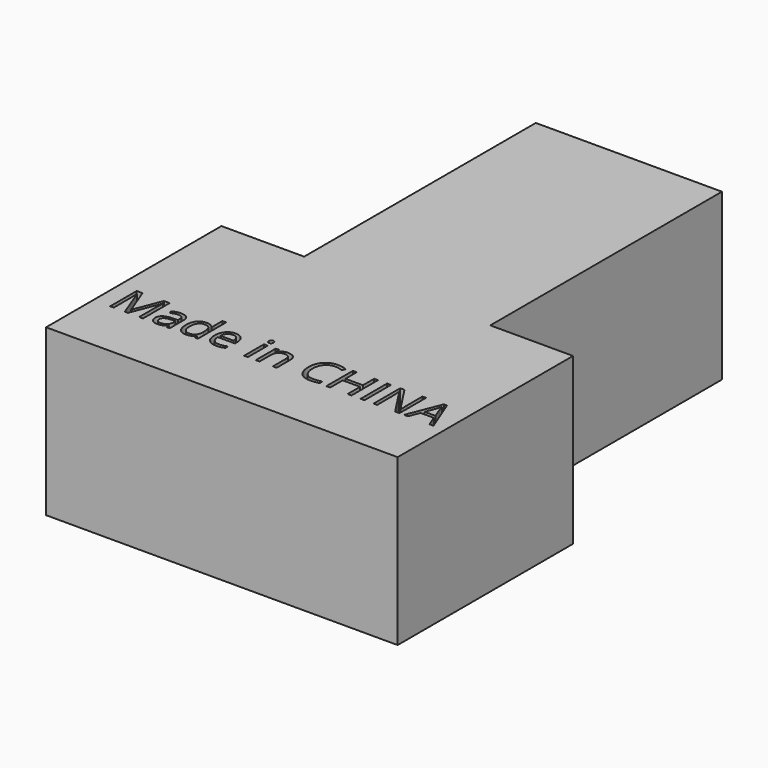
from build123d import *

# Parameters (mm, degrees)
F0_W         = 2.3149197708
F0_H         = 15.276686349
F0_W_2       = 2.3684439274
F0_H_2       = 20.3793226068
F0_W_3       = 114.3
F0_H_3       = 177.8
F0_TEXT_SIZE = 28.5462168273
F1_DEPTH     = 101.6
F2_DEPTH     = 254


# Not quite as in the source:
# - Text() gives the source's letters only with a copy of the font that has no kerning and outlines rounded to 1/6400 em; it was checked with that copy


with BuildPart() as f1:
    # F0 (on Top) → F1 (new body)
    with BuildSketch(Plane.XY):
        Polygon((-51.415306741, 48.4471506375), (-102.215306741, 48.4471506375), (-102.215306741, -86.1728493625), (113.684693259, -86.1728493625), (113.684693259, 48.4471506375), (62.884693259, 48.4471506375), align=None)
        with BuildLine():
            Line((-80.9077623426, -49.9574655533), (-82.816790593, -49.9574655533))
            Line((-82.816790593, -49.9574655533), (-89.7303274808, -31.8930627173))
            Line((-89.7303274808, -31.8930627173), (-89.8418361403, -31.8930627173))
            add(Edge.make_bspline(
                [(-89.8418361403, -31.8930627173), (-89.6455808996, -34.0384893257), (-89.6455808996, -36.9956989751)],
                knots=[0, 0, 0, 1, 1, 1], degree=2))
            Line((-89.6455808996, -36.9956989751), (-89.6455808996, -49.9574655533))
            Line((-89.6455808996, -49.9574655533), (-91.8356109718, -49.9574655533))
            Line((-91.8356109718, -49.9574655533), (-91.8356109718, -29.5781429464))
            Line((-91.8356109718, -29.5781429464), (-88.2673338684, -29.5781429464))
            Line((-88.2673338684, -29.5781429464), (-81.8132126576, -46.3891884499))
            Line((-81.8132126576, -46.3891884499), (-81.7017039981, -46.3891884499))
            Line((-81.7017039981, -46.3891884499), (-75.1940586308, -29.5781429464))
            Line((-75.1940586308, -29.5781429464), (-71.6525436057, -29.5781429464))
            Line((-71.6525436057, -29.5781429464), (-71.6525436057, -49.9574655533))
            Line((-71.6525436057, -49.9574655533), (-74.0209875331, -49.9574655533))
            Line((-74.0209875331, -49.9574655533), (-74.0209875331, -36.8262058127))
            add(Edge.make_bspline(
                [(-74.0209875331, -36.8262058127), (-74.0209875331, -34.5692705448), (-73.8247322924, -31.9198247955)],
                knots=[0, 0, 0, 1, 1, 1], degree=2))
            Line((-73.8247322924, -31.9198247955), (-73.9362409518, -31.9198247955))
            Line((-73.9362409518, -31.9198247955), (-80.9077623426, -49.9574655533))
        make_face(mode=Mode.SUBTRACT)
        with BuildLine():
            Line((-55.3009137793, -49.9574655533), (-57.0181471353, -49.9574655533))
            Line((-57.0181471353, -49.9574655533), (-57.4775628124, -47.7808165202))
            Line((-57.4775628124, -47.7808165202), (-57.5890714719, -47.7808165202))
            add(Edge.make_bspline(
                [(-57.5890714719, -47.7808165202), (-58.7309201449, -49.2170480543), (-59.8660782985, -49.7277577147)],
                knots=[0, 0, 0, 1, 1, 1], degree=2))
            add(Edge.make_bspline(
                [(-59.8660782985, -49.7277577147), (-61.001236452, -50.2384673752), (-62.7050887689, -50.2384673752)],
                knots=[0, 0, 0, 1, 1, 1], degree=2))
            add(Edge.make_bspline(
                [(-62.7050887689, -50.2384673752), (-64.9754050759, -50.2384673752), (-66.2644451795, -49.0653962774)],
                knots=[0, 0, 0, 1, 1, 1], degree=2))
            add(Edge.make_bspline(
                [(-66.2644451795, -49.0653962774), (-67.5534852831, -47.8923251797), (-67.5534852831, -45.7335175321)],
                knots=[0, 0, 0, 1, 1, 1], degree=2))
            add(Edge.make_bspline(
                [(-67.5534852831, -45.7335175321), (-67.5534852831, -41.1081383368), (-60.1537706399, -40.8851210178)],
                knots=[0, 0, 0, 1, 1, 1], degree=2))
            Line((-60.1537706399, -40.8851210178), (-57.5623093936, -40.8003744366))
            Line((-57.5623093936, -40.8003744366), (-57.5623093936, -39.8503206579))
            add(Edge.make_bspline(
                [(-57.5623093936, -39.8503206579), (-57.5623093936, -38.052801067), (-58.3339493172, -37.1964145622)],
                knots=[0, 0, 0, 1, 1, 1], degree=2))
            add(Edge.make_bspline(
                [(-58.3339493172, -37.1964145622), (-59.1055892408, -36.3400280574), (-60.8094415577, -36.3400280574)],
                knots=[0, 0, 0, 1, 1, 1], degree=2))
            add(Edge.make_bspline(
                [(-60.8094415577, -36.3400280574), (-62.718469808, -36.3400280574), (-65.1270568528, -37.5086388087)],
                knots=[0, 0, 0, 1, 1, 1], degree=2))
            Line((-65.1270568528, -37.5086388087), (-65.8407122735, -35.7378812962))
            add(Edge.make_bspline(
                [(-65.8407122735, -35.7378812962), (-64.7122446395, -35.1268138422), (-63.3674502062, -34.7789068246)],
                knots=[0, 0, 0, 1, 1, 1], degree=2))
            add(Edge.make_bspline(
                [(-63.3674502062, -34.7789068246), (-62.0226557728, -34.4309998071), (-60.6667104735, -34.4309998071)],
                knots=[0, 0, 0, 1, 1, 1], degree=2))
            add(Edge.make_bspline(
                [(-60.6667104735, -34.4309998071), (-57.9369784894, -34.4309998071), (-56.6189461344, -35.641983849)],
                knots=[0, 0, 0, 1, 1, 1], degree=2))
            add(Edge.make_bspline(
                [(-56.6189461344, -35.641983849), (-55.3009137793, -36.852967891), (-55.3009137793, -39.5291757186)],
                knots=[0, 0, 0, 1, 1, 1], degree=2))
            Line((-55.3009137793, -39.5291757186), (-55.3009137793, -49.9574655533))
        make_face(mode=Mode.SUBTRACT)
        with BuildLine():
            Line((-39.832432536, -49.9574655533), (-40.1401964362, -47.9101665652))
            Line((-40.1401964362, -47.9101665652), (-40.2650861348, -47.9101665652))
            add(Edge.make_bspline(
                [(-40.2650861348, -47.9101665652), (-41.866350485, -50.2384673752), (-45.0599584925, -50.2384673752)],
                knots=[0, 0, 0, 1, 1, 1], degree=2))
            add(Edge.make_bspline(
                [(-45.0599584925, -50.2384673752), (-48.0573112594, -50.2384673752), (-49.723250632, -48.1889382139)],
                knots=[0, 0, 0, 1, 1, 1], degree=2))
            add(Edge.make_bspline(
                [(-49.723250632, -48.1889382139), (-51.3891900047, -46.1394090526), (-51.3891900047, -42.3614956694)],
                knots=[0, 0, 0, 1, 1, 1], degree=2))
            add(Edge.make_bspline(
                [(-51.3891900047, -42.3614956694), (-51.3891900047, -38.5835822861), (-49.7165601125, -36.4916798343)],
                knots=[0, 0, 0, 1, 1, 1], degree=2))
            add(Edge.make_bspline(
                [(-49.7165601125, -36.4916798343), (-48.0439302202, -34.3997773824), (-45.0599584925, -34.3997773824)],
                knots=[0, 0, 0, 1, 1, 1], degree=2))
            add(Edge.make_bspline(
                [(-45.0599584925, -34.3997773824), (-41.9510970662, -34.3997773824), (-40.2918482131, -36.6611729967)],
                knots=[0, 0, 0, 1, 1, 1], degree=2))
            Line((-40.2918482131, -36.6611729967), (-40.1089740115, -36.6611729967))
            Line((-40.1089740115, -36.6611729967), (-40.2071016319, -35.559467441))
            Line((-40.2071016319, -35.559467441), (-40.2650861348, -34.4845239636))
            Line((-40.2650861348, -34.4845239636), (-40.2650861348, -28.2668011109))
            Line((-40.2650861348, -28.2668011109), (-37.950166364, -28.2668011109))
            Line((-37.950166364, -28.2668011109), (-37.950166364, -49.9574655533))
            Line((-37.950166364, -49.9574655533), (-39.832432536, -49.9574655533))
        make_face(mode=Mode.SUBTRACT)
        with BuildLine():
            add(Edge.make_bspline(
                [(-23.9491390795, -50.0065293634), (-25.0419239424, -50.2384673752), (-26.589664136, -50.2384673752)],
                knots=[0, 0, 0, 1, 1, 1], degree=2))
            add(Edge.make_bspline(
                [(-26.589664136, -50.2384673752), (-29.9750670379, -50.2384673752), (-31.9353892715, -48.1733270016)],
                knots=[0, 0, 0, 1, 1, 1], degree=2))
            add(Edge.make_bspline(
                [(-31.9353892715, -48.1733270016), (-33.8957115052, -46.108186628), (-33.8957115052, -42.4462422506)],
                knots=[0, 0, 0, 1, 1, 1], degree=2))
            add(Edge.make_bspline(
                [(-33.8957115052, -42.4462422506), (-33.8957115052, -38.7486151022), (-32.0758901825, -36.5741962423)],
                knots=[0, 0, 0, 1, 1, 1], degree=2))
            add(Edge.make_bspline(
                [(-32.0758901825, -36.5741962423), (-30.2560688597, -34.3997773824), (-27.1873505508, -34.3997773824)],
                knots=[0, 0, 0, 1, 1, 1], degree=2))
            add(Edge.make_bspline(
                [(-27.1873505508, -34.3997773824), (-24.3193478289, -34.3997773824), (-22.6467179367, -36.288734074)],
                knots=[0, 0, 0, 1, 1, 1], degree=2))
            add(Edge.make_bspline(
                [(-22.6467179367, -36.288734074), (-20.9740880445, -38.1776907656), (-20.9740880445, -41.2731711528)],
                knots=[0, 0, 0, 1, 1, 1], degree=2))
            Line((-20.9740880445, -41.2731711528), (-20.9740880445, -42.7361647652))
            Line((-20.9740880445, -42.7361647652), (-31.4960451532, -42.7361647652))
            add(Edge.make_bspline(
                [(-31.4960451532, -42.7361647652), (-31.4246796111, -45.4257536319), (-30.1356395075, -46.8196118755)],
                knots=[0, 0, 0, 1, 1, 1], degree=2))
            add(Edge.make_bspline(
                [(-30.1356395075, -46.8196118755), (-28.8465994039, -48.213470119), (-26.5049175548, -48.213470119)],
                knots=[0, 0, 0, 1, 1, 1], degree=2))
            add(Edge.make_bspline(
                [(-26.5049175548, -48.213470119), (-24.0383460071, -48.213470119), (-21.6297589623, -47.1831301054)],
                knots=[0, 0, 0, 1, 1, 1], degree=2))
            Line((-21.6297589623, -47.1831301054), (-21.6297589623, -49.248270479))
            add(Edge.make_bspline(
                [(-21.6297589623, -49.248270479), (-22.8563542166, -49.7745913517), (-23.9491390795, -50.0065293634)],
                knots=[0, 0, 0, 1, 1, 1], degree=2))
        make_face(mode=Mode.SUBTRACT)
        with Locations((-8.4516655847, -42.3191223788)):
            Rectangle(F0_W, F0_H, mode=Mode.SUBTRACT)
        with BuildLine():
            add(Edge.make_bspline(
                [(-9.4151004026, -31.7057281693), (-9.8053807108, -31.3221383807), (-9.8053807108, -30.5415777643)],
                knots=[0, 0, 0, 1, 1, 1], degree=2))
            add(Edge.make_bspline(
                [(-9.8053807108, -30.5415777643), (-9.8053807108, -29.7476361088), (-9.4151004026, -29.3774273594)],
                knots=[0, 0, 0, 1, 1, 1], degree=2))
            add(Edge.make_bspline(
                [(-9.4151004026, -29.3774273594), (-9.0248200945, -29.0072186099), (-8.4360543724, -29.0072186099)],
                knots=[0, 0, 0, 1, 1, 1], degree=2))
            add(Edge.make_bspline(
                [(-8.4360543724, -29.0072186099), (-7.878511075, -29.0072186099), (-7.4748497277, -29.3841178789)],
                knots=[0, 0, 0, 1, 1, 1], degree=2))
            add(Edge.make_bspline(
                [(-7.4748497277, -29.3841178789), (-7.0711883803, -29.761017148), (-7.0711883803, -30.5415777643)],
                knots=[0, 0, 0, 1, 1, 1], degree=2))
            add(Edge.make_bspline(
                [(-7.0711883803, -30.5415777643), (-7.0711883803, -31.3221383807), (-7.4748497277, -31.7057281693)],
                knots=[0, 0, 0, 1, 1, 1], degree=2))
            add(Edge.make_bspline(
                [(-7.4748497277, -31.7057281693), (-7.878511075, -32.0893179579), (-8.4360543724, -32.0893179579)],
                knots=[0, 0, 0, 1, 1, 1], degree=2))
            add(Edge.make_bspline(
                [(-8.4360543724, -32.0893179579), (-9.0248200945, -32.0893179579), (-9.4151004026, -31.7057281693)],
                knots=[0, 0, 0, 1, 1, 1], degree=2))
        make_face(mode=Mode.SUBTRACT)
        with BuildLine():
            Line((10.3821470017, -49.9574655533), (8.0672272309, -49.9574655533))
            Line((8.0672272309, -49.9574655533), (8.0672272309, -40.0733379768))
            add(Edge.make_bspline(
                [(8.0672272309, -40.0733379768), (8.0672272309, -38.2089131903), (7.2175312456, -37.287851663)],
                knots=[0, 0, 0, 1, 1, 1], degree=2))
            add(Edge.make_bspline(
                [(7.2175312456, -37.287851663), (6.3678352604, -36.3667901357), (4.552474284, -36.3667901357)],
                knots=[0, 0, 0, 1, 1, 1], degree=2))
            add(Edge.make_bspline(
                [(4.552474284, -36.3667901357), (2.1572682783, -36.3667901357), (1.0421816835, -37.6625207588)],
                knots=[0, 0, 0, 1, 1, 1], degree=2))
            add(Edge.make_bspline(
                [(1.0421816835, -37.6625207588), (-0.0729049113, -38.958251382), (-0.0729049113, -41.9422231097)],
                knots=[0, 0, 0, 1, 1, 1], degree=2))
            Line((-0.0729049113, -41.9422231097), (-0.0729049113, -49.9574655533))
            Line((-0.0729049113, -49.9574655533), (-2.3878246821, -49.9574655533))
            Line((-2.3878246821, -49.9574655533), (-2.3878246821, -34.6807792043))
            Line((-2.3878246821, -34.6807792043), (-0.5055585101, -34.6807792043))
            Line((-0.5055585101, -34.6807792043), (-0.1308894142, -36.7726816562))
            Line((-0.1308894142, -36.7726816562), (-0.0193807547, -36.7726816562))
            add(Edge.make_bspline(
                [(-0.0193807547, -36.7726816562), (0.6942746659, -35.6442140222), (1.97662425, -35.0219957023)],
                knots=[0, 0, 0, 1, 1, 1], degree=2))
            add(Edge.make_bspline(
                [(1.97662425, -35.0219957023), (3.258973834, -34.3997773824), (4.8334761059, -34.3997773824)],
                knots=[0, 0, 0, 1, 1, 1], degree=2))
            add(Edge.make_bspline(
                [(4.8334761059, -34.3997773824), (7.5944305147, -34.3997773824), (8.9882887582, -35.7311907766)],
                knots=[0, 0, 0, 1, 1, 1], degree=2))
            add(Edge.make_bspline(
                [(8.9882887582, -35.7311907766), (10.3821470017, -37.0626041708), (10.3821470017, -39.993051742)],
                knots=[0, 0, 0, 1, 1, 1], degree=2))
            Line((10.3821470017, -39.993051742), (10.3821470017, -49.9574655533))
        make_face(mode=Mode.SUBTRACT)
        with BuildLine():
            add(Edge.make_bspline(
                [(36.2521560014, -32.4907491321), (33.9372362306, -31.4068849619), (31.6223164597, -31.4068849619)],
                knots=[0, 0, 0, 1, 1, 1], degree=2))
            add(Edge.make_bspline(
                [(31.6223164597, -31.4068849619), (28.2636756362, -31.4068849619), (26.3189646148, -33.6437486711)],
                knots=[0, 0, 0, 1, 1, 1], degree=2))
            add(Edge.make_bspline(
                [(26.3189646148, -33.6437486711), (24.3742535934, -35.8806123803), (24.3742535934, -39.770034423)],
                knots=[0, 0, 0, 1, 1, 1], degree=2))
            add(Edge.make_bspline(
                [(24.3742535934, -39.770034423), (24.3742535934, -43.7665047788), (26.2498292459, -45.9498443315)],
                knots=[0, 0, 0, 1, 1, 1], degree=2))
            add(Edge.make_bspline(
                [(26.2498292459, -45.9498443315), (28.1254048984, -48.1331838841), (31.5955543815, -48.1331838841)],
                knots=[0, 0, 0, 1, 1, 1], degree=2))
            add(Edge.make_bspline(
                [(31.5955543815, -48.1331838841), (33.7275999508, -48.1331838841), (36.4617922812, -47.3660043069)],
                knots=[0, 0, 0, 1, 1, 1], degree=2))
            Line((36.4617922812, -47.3660043069), (36.4617922812, -49.4400653733))
            add(Edge.make_bspline(
                [(36.4617922812, -49.4400653733), (34.3431277511, -50.2384673752), (31.2342663247, -50.2384673752)],
                knots=[0, 0, 0, 1, 1, 1], degree=2))
            add(Edge.make_bspline(
                [(31.2342663247, -50.2384673752), (26.7337768281, -50.2384673752), (24.287276839, -47.5042750447)],
                knots=[0, 0, 0, 1, 1, 1], degree=2))
            add(Edge.make_bspline(
                [(24.287276839, -47.5042750447), (21.84077685, -44.7700827142), (21.84077685, -39.7388119984)],
                knots=[0, 0, 0, 1, 1, 1], degree=2))
            add(Edge.make_bspline(
                [(21.84077685, -39.7388119984), (21.84077685, -36.5898074546), (23.0183082941, -34.2213635272)],
                knots=[0, 0, 0, 1, 1, 1], degree=2))
            add(Edge.make_bspline(
                [(23.0183082941, -34.2213635272), (24.1958397383, -31.8529195998), (26.4193224083, -30.5705700158)],
                knots=[0, 0, 0, 1, 1, 1], degree=2))
            add(Edge.make_bspline(
                [(26.4193224083, -30.5705700158), (28.6428050784, -29.2882204318), (31.6535388844, -29.2882204318)],
                knots=[0, 0, 0, 1, 1, 1], degree=2))
            add(Edge.make_bspline(
                [(31.6535388844, -29.2882204318), (34.8560675847, -29.2882204318), (37.2557339368, -30.4568311831)],
                knots=[0, 0, 0, 1, 1, 1], degree=2))
            Line((37.2557339368, -30.4568311831), (36.2521560014, -32.4907491321))
        make_face(mode=Mode.SUBTRACT)
        Polygon((56.381699211, -29.5781429464), (56.381699211, -49.9574655533), (54.0132552836, -49.9574655533), (54.0132552836, -40.3677208379), (43.2772015488, -40.3677208379), (43.2772015488, -49.9574655533), (40.9087576214, -49.9574655533), (40.9087576214, -29.5781429464), (43.2772015488, -29.5781429464), (43.2772015488, -38.2490563077), (54.0132552836, -38.2490563077), (54.0132552836, -29.5781429464), align=None, mode=Mode.SUBTRACT)
        with Locations((63.1547351879, -39.7678042498)):
            Rectangle(F0_W_2, F0_H_2, mode=Mode.SUBTRACT)
        with BuildLine():
            Line((85.8467473924, -29.5781429464), (85.8467473924, -49.9574655533))
            Line((85.8467473924, -49.9574655533), (83.1437774866, -49.9574655533))
            Line((83.1437774866, -49.9574655533), (72.0062925776, -32.8564975352))
            Line((72.0062925776, -32.8564975352), (71.8947839181, -32.8564975352))
            add(Edge.make_bspline(
                [(71.8947839181, -32.8564975352), (72.1178012371, -35.8672313412), (72.1178012371, -38.3739460063)],
                knots=[0, 0, 0, 1, 1, 1], degree=2))
            Line((72.1178012371, -38.3739460063), (72.1178012371, -49.9574655533))
            Line((72.1178012371, -49.9574655533), (69.9277711648, -49.9574655533))
            Line((69.9277711648, -49.9574655533), (69.9277711648, -29.5781429464))
            Line((69.9277711648, -29.5781429464), (72.6039789924, -29.5781429464))
            Line((72.6039789924, -29.5781429464), (83.7147018231, -46.6122057688))
            Line((83.7147018231, -46.6122057688), (83.8262104826, -46.6122057688))
            add(Edge.make_bspline(
                [(83.8262104826, -46.6122057688), (83.7994484043, -46.237536673), (83.701320784, -44.1946980313)],
                knots=[0, 0, 0, 1, 1, 1], degree=2))
            add(Edge.make_bspline(
                [(83.701320784, -44.1946980313), (83.6031931637, -42.1518593896), (83.6299552419, -41.2731711528)],
                knots=[0, 0, 0, 1, 1, 1], degree=2))
            Line((83.6299552419, -41.2731711528), (83.6299552419, -29.5781429464))
            Line((83.6299552419, -29.5781429464), (85.8467473924, -29.5781429464))
        make_face(mode=Mode.SUBTRACT)
        Polygon((106.7122477546, -49.9574655533), (104.259057246, -49.9574655533), (101.7211201562, -43.4765822642), (93.5542259358, -43.4765822642), (91.0475112706, -49.9574655533), (88.6478449186, -49.9574655533), (96.7032304795, -29.4933963652), (98.6970053111, -29.4933963652), align=None, mode=Mode.SUBTRACT)
        with Locations((5.734693259, 137.3471506375)):
            Rectangle(F0_W_3, F0_H_3)
        with BuildLine():
            add(Edge.make_bspline(
                [(-47.9168103484, -46.8062308363), (-46.8440970442, -48.2982167002), (-44.7655756315, -48.2982167002)],
                knots=[0, 0, 0, 1, 1, 1], degree=2))
            add(Edge.make_bspline(
                [(-44.7655756315, -48.2982167002), (-42.3971317041, -48.2982167002), (-41.3311089195, -47.0091765966)],
                knots=[0, 0, 0, 1, 1, 1], degree=2))
            add(Edge.make_bspline(
                [(-41.3311089195, -47.0091765966), (-40.2650861348, -45.720136493), (-40.2650861348, -42.8476734247)],
                knots=[0, 0, 0, 1, 1, 1], degree=2))
            Line((-40.2650861348, -42.8476734247), (-40.2650861348, -42.3614956694))
            add(Edge.make_bspline(
                [(-40.2650861348, -42.3614956694), (-40.2650861348, -39.1143635053), (-41.3444899586, -37.7271957813)],
                knots=[0, 0, 0, 1, 1, 1], degree=2))
            add(Edge.make_bspline(
                [(-41.3444899586, -37.7271957813), (-42.4238937824, -36.3400280574), (-44.7923377098, -36.3400280574)],
                knots=[0, 0, 0, 1, 1, 1], degree=2))
            add(Edge.make_bspline(
                [(-44.7923377098, -36.3400280574), (-46.8307160051, -36.3400280574), (-47.9101198289, -37.9212208488)],
                knots=[0, 0, 0, 1, 1, 1], degree=2))
            add(Edge.make_bspline(
                [(-47.9101198289, -37.9212208488), (-48.9895236526, -39.5024136403), (-48.9895236526, -42.3882577477)],
                knots=[0, 0, 0, 1, 1, 1], degree=2))
            add(Edge.make_bspline(
                [(-48.9895236526, -42.3882577477), (-48.9895236526, -45.3142449725), (-47.9168103484, -46.8062308363)],
                knots=[0, 0, 0, 1, 1, 1], degree=2))
        make_face()
        with BuildLine():
            add(Edge.make_bspline(
                [(-64.3687979683, -47.6715380339), (-63.6105390839, -48.3249787785), (-62.2456730918, -48.3249787785)],
                knots=[0, 0, 0, 1, 1, 1], degree=2))
            add(Edge.make_bspline(
                [(-62.2456730918, -48.3249787785), (-60.0824050979, -48.3249787785), (-58.849119324, -47.1407568148)],
                knots=[0, 0, 0, 1, 1, 1], degree=2))
            add(Edge.make_bspline(
                [(-58.849119324, -47.1407568148), (-57.6158335501, -45.9565348511), (-57.6158335501, -43.8244892818)],
                knots=[0, 0, 0, 1, 1, 1], degree=2))
            Line((-57.6158335501, -43.8244892818), (-57.6158335501, -42.4462422506))
            Line((-57.6158335501, -42.4462422506), (-59.930753321, -42.5399095246))
            add(Edge.make_bspline(
                [(-59.930753321, -42.5399095246), (-62.6917077297, -42.6380371449), (-63.9093822913, -43.3985262026)],
                knots=[0, 0, 0, 1, 1, 1], degree=2))
            add(Edge.make_bspline(
                [(-63.9093822913, -43.3985262026), (-65.1270568528, -44.1590152602), (-65.1270568528, -45.7602796104)],
                knots=[0, 0, 0, 1, 1, 1], degree=2))
            add(Edge.make_bspline(
                [(-65.1270568528, -45.7602796104), (-65.1270568528, -47.0180972893), (-64.3687979683, -47.6715380339)],
                knots=[0, 0, 0, 1, 1, 1], degree=2))
        make_face()
        with BuildLine():
            Line((94.3927710551, -41.3445366949), (100.9851630036, -41.3445366949))
            Line((100.9851630036, -41.3445366949), (98.6122587299, -35.0286862219))
            add(Edge.make_bspline(
                [(98.6122587299, -35.0286862219), (98.1528430528, -33.8288530459), (97.6666652975, -32.0893179579)],
                knots=[0, 0, 0, 1, 1, 1], degree=2))
            add(Edge.make_bspline(
                [(97.6666652975, -32.0893179579), (97.3589013973, -33.4274218717), (96.7879770608, -35.0286862219)],
                knots=[0, 0, 0, 1, 1, 1], degree=2))
            Line((96.7879770608, -35.0286862219), (94.3927710551, -41.3445366949))
        make_face()
        with BuildLine():
            add(Edge.make_bspline(
                [(-24.4286263152, -37.5041784624), (-25.4032119991, -36.3400280574), (-27.2185729755, -36.3400280574)],
                knots=[0, 0, 0, 1, 1, 1], degree=2))
            add(Edge.make_bspline(
                [(-27.2185729755, -36.3400280574), (-29.0562356837, -36.3400280574), (-30.1512507198, -37.5376310602)],
                knots=[0, 0, 0, 1, 1, 1], degree=2))
            add(Edge.make_bspline(
                [(-30.1512507198, -37.5376310602), (-31.2462657559, -38.735234063), (-31.4425209966, -40.8538985932)],
                knots=[0, 0, 0, 1, 1, 1], degree=2))
            Line((-31.4425209966, -40.8538985932), (-23.4540406314, -40.8538985932))
            add(Edge.make_bspline(
                [(-23.4540406314, -40.8538985932), (-23.4540406314, -38.6683288674), (-24.4286263152, -37.5041784624)],
                knots=[0, 0, 0, 1, 1, 1], degree=2))
        make_face()
        with Locations((-94.636708498, -49.9574655533)):
            Text('Made in CHINA', F0_TEXT_SIZE, font='Open Sans', text_align=(TextAlign.LEFT, TextAlign.BOTTOM))
    extrude(amount=F1_DEPTH)

    # F0 (on Top) → F2 (cut)
    with BuildSketch(Plane.XY):
        with Locations((-94.636708498, -49.9574655533)):
            Text('Made in CHINA', F0_TEXT_SIZE, font='Open Sans', text_align=(TextAlign.LEFT, TextAlign.BOTTOM))
    extrude(amount=F2_DEPTH, mode=Mode.SUBTRACT)


solid = f1.part
